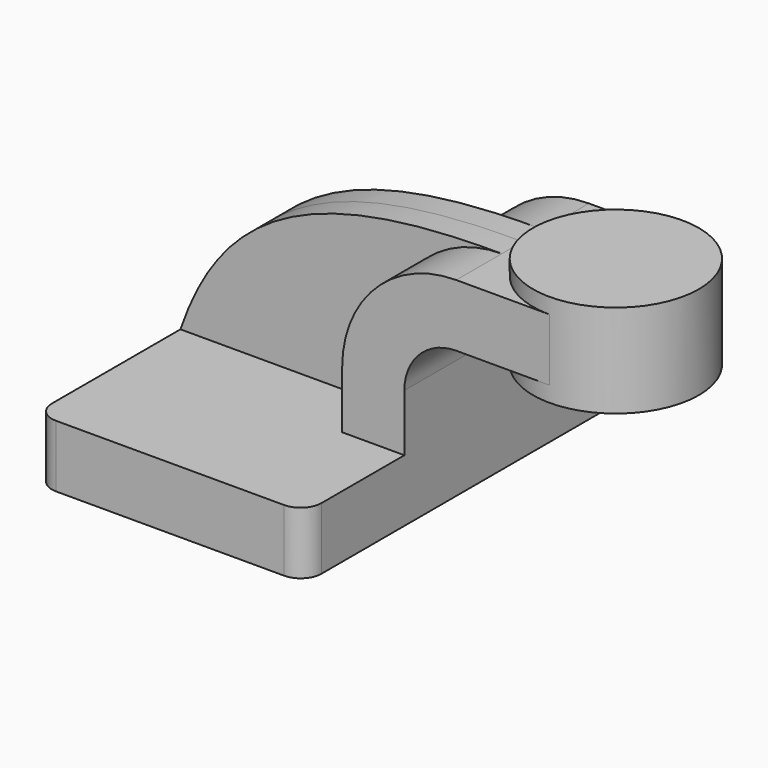
from build123d import *

# Parameters (mm, degrees)
F1_DEPTH = 63.5
F2_DEPTH = 25.4
F3_DEPTH = 7.9375
F0_W     = 25.4
F0_H     = 19.05
F4_DEPTH = 25.4
F6_R     = 6.35


# Not quite as in the source:
# - a feature names something its author has since deleted; it is built from what else it names


with BuildPart() as f1:
    # F0 (on Front) → F1 (new body, symmetric)
    with BuildSketch(Plane.XZ):
        Polygon((22.225, 9.525), (-41.275, 9.525), (-41.275, -9.525), (41.275, -9.525), (41.275, 9.525), align=None)
    extrude(amount=F1_DEPTH, both=True)

    # F0 (on Front) → F2 (join, symmetric)
    with BuildSketch(Plane.XZ):
        with BuildLine():
            Line((22.225, 27.0002), (22.225, 9.525))
            Line((22.225, 9.525), (41.275, 9.525))
            Line((41.275, 9.525), (41.275, 27.0002))
            ThreePointArc((41.275, 27.0002), (45.9246798487, 38.2255201513), (57.15, 42.8752))
            Line((57.15, 42.8752), (60.325, 42.8752))
            Line((60.325, 42.8752), (60.325, 61.9252))
            Line((60.325, 61.9252), (57.15, 61.9252))
            ThreePointArc((57.15, 61.9252), (32.4542956671, 51.6959043329), (22.225, 27.0002))
        make_face()
    extrude(amount=F2_DEPTH, both=True)

    # F0 (on Front) → F3 (join, symmetric)
    with BuildSketch(Plane.XZ):
        with BuildLine():
            add(Edge.make_bspline(
                [(-41.275, 9.525), (-28.3377878368, 47.713726759), (0, 62.2769519687), (57.15, 61.9252)],
                knots=[0, 0, 0, 0, 111.5045361635, 111.5045361635, 111.5045361635, 111.5045361635], degree=3))
            Line((-41.275, 9.525), (22.225, 9.525))
            Line((22.225, 9.525), (22.225, 27.0002))
            ThreePointArc((22.225, 27.0002), (32.4542956671, 51.6959043329), (57.15, 61.9252))
        make_face()
    extrude(amount=F3_DEPTH, both=True)

    # F0 (on Front) → F4 (join, symmetric)
    with BuildSketch(Plane.XZ):
        with Locations((73.025, 52.4002)):
            Rectangle(F0_W, F0_H)
    extrude(amount=F4_DEPTH, both=True)

    # F0 (on Front) → F5 (revolve)
    with BuildSketch(Plane.XZ):
        Polygon((85.725, 66.675), (85.725, 61.9252), (85.725, 42.8752), (85.725, 38.1), (111.125, 38.1), (111.125, 66.675), align=None)
    revolve(axis=Axis((85.725, 0, 52.3875), (0, 0, -1)))

    # F6
    f6_edges = [f1.edges().sort_by_distance(p)[0] for p in [
        (-41.275, -63.5, 0),
        (41.275, -63.5, 0),
        (41.275, 63.5, 0),
        (-41.275, 63.5, 0),
    ]]
    fillet(f6_edges, radius=F6_R)


solid = f1.part
